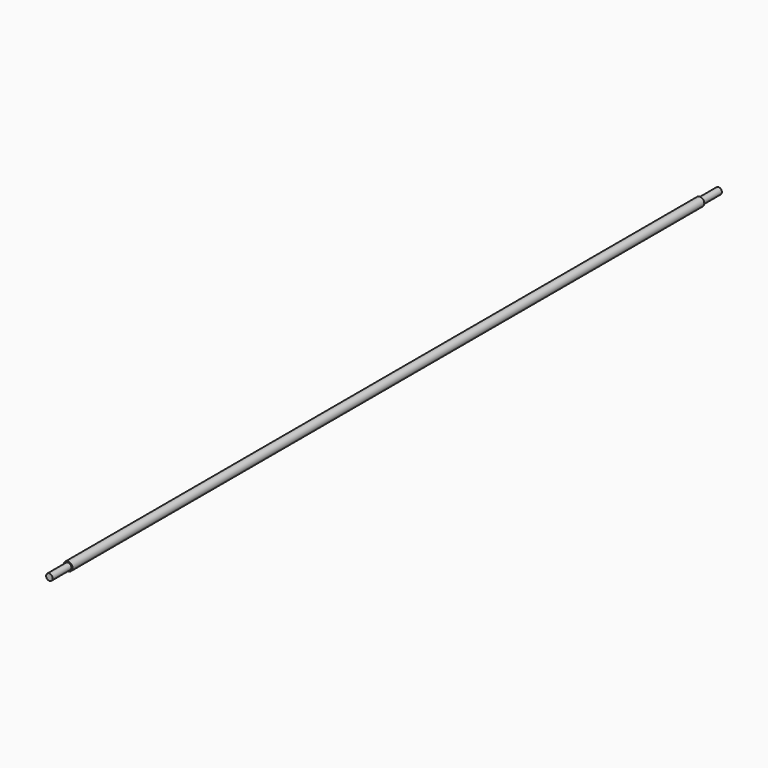
from build123d import *

# Parameters (mm, degrees)
F0_R          = 9.525
F0_R_2        = 7.14375
F1_DEPTH      = 855.98
F1_DEPTH_BACK = 855.98
F2_R          = 7.14375
F3_DEPTH      = 906.78
F3_DEPTH_BACK = 906.78


# Not quite as in the source:
# - a feature names something its author has since deleted; it is built from what else it names


with BuildPart() as f1:
    # F0 (on Front) → F1 (new body, two sides)
    with BuildSketch(Plane.XZ) as f1_sk:
        Circle(F0_R)
        Circle(F0_R_2, mode=Mode.SUBTRACT)
    extrude(amount=F1_DEPTH)
    extrude(f1_sk.sketch, amount=-F1_DEPTH_BACK)

    # F2 (on Front) → F3 (join, two sides)
    with BuildSketch(Plane.XZ) as f3_sk:
        Circle(F2_R)
    extrude(amount=F3_DEPTH)
    extrude(f3_sk.sketch, amount=-F3_DEPTH_BACK)


solid = f1.part
